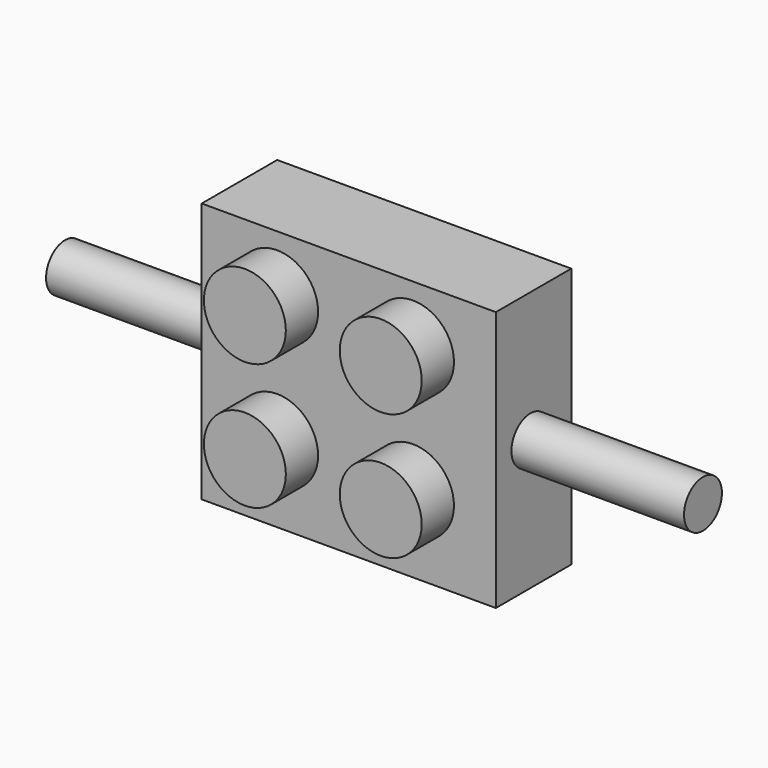
from build123d import *

# Parameters (mm, degrees)
F0_R      = 7.8435703096
F1_DEPTH  = 5.67
F0_R_2    = 7.7757185056
F2_W      = 17.6903378959
F2_H      = 15.67
F3_DEPTH  = 5.67
F4_R      = 1.425
F5_DEPTH  = 10.38
F6_R      = 1.425
F7_DEPTH  = 10.38
F8_R      = 2.465
F9_DEPTH  = 2.425
F10_W     = 12.8629952669
F10_H     = 10.9573621303
F11_DEPTH = 3
F12_R     = 2.75
F12_R_2   = 1.75
F13_DEPTH = 2
F14_R     = 4.345
F14_R_2   = 3.4662678384
F15_DEPTH = 25
F14_R_3   = 3.1273613379
F14_R_4   = 4.1038801884
F14_R_5   = 4.2870364602
F16_DEPTH = 25


with BuildPart() as f1:
    # F0 (on Front) → F1 (new body)
    with BuildSketch(Plane.XZ):
        with Locations((-31.0182443455, 13.5022135742)):
            Circle(F0_R)
    extrude(amount=F1_DEPTH)

    # F14 (on Front) → F15, piece 2 (join)
    with BuildSketch(Plane.XZ):
        with Locations((-31.2459040433, 14.0220327303)):
            Circle(F14_R)
        with Locations((-31.2459040433, 14.0220327303)):
            Circle(F14_R_3, mode=Mode.SUBTRACT)
    extrude(amount=F15_DEPTH)

    # F14 (on Front) → F16 (cut)
    with BuildSketch(Plane.XZ):
        with Locations((27.6749636978, 13.738758862)):
            Circle(F14_R)
        with Locations((27.6749636978, 13.738758862)):
            Circle(F14_R_2, mode=Mode.SUBTRACT)
        with Locations((-30.9626311064, -35.5508103967)):
            Circle(F14_R)
        with Locations((-30.9626311064, -35.5508103967)):
            Circle(F14_R_4, mode=Mode.SUBTRACT)
        with Locations((27.9582366347, -35.5508103967)):
            Circle(F14_R)
        with Locations((27.9582366347, -35.5508103967)):
            Circle(F14_R_5, mode=Mode.SUBTRACT)
        with Locations((-31.2459040433, 14.0220327303)):
            Circle(F14_R)
        with Locations((-31.2459040433, 14.0220327303)):
            Circle(F14_R_3, mode=Mode.SUBTRACT)
    extrude(amount=-F16_DEPTH, mode=Mode.SUBTRACT)


with BuildPart() as f1b:
    # F0 (on Front) → F1, piece 2 (new body)
    with BuildSketch(Plane.XZ):
        with Locations((27.6562659057, 13.5022135742)):
            Circle(F0_R_2)
    extrude(amount=F1_DEPTH)

    # F14 (on Front) → F15 (join)
    with BuildSketch(Plane.XZ):
        with Locations((27.6749636978, 13.738758862)):
            Circle(F14_R)
        with Locations((27.6749636978, 13.738758862)):
            Circle(F14_R_2, mode=Mode.SUBTRACT)
    extrude(amount=F15_DEPTH)


with BuildPart() as f1c:
    # F0 (on Front) → F1, piece 3 (new body)
    with BuildSketch(Plane.XZ):
        with Locations((-31.0182443455, -35.7866174178)):
            Circle(F0_R_2)
    extrude(amount=F1_DEPTH)

    # F14 (on Front) → F15, piece 3 (join)
    with BuildSketch(Plane.XZ):
        with Locations((-30.9626311064, -35.5508103967)):
            Circle(F14_R)
        with Locations((-30.9626311064, -35.5508103967)):
            Circle(F14_R_4, mode=Mode.SUBTRACT)
    extrude(amount=F15_DEPTH)


with BuildPart() as f1d:
    # F0 (on Front) → F1, piece 4 (new body)
    with BuildSketch(Plane.XZ):
        with Locations((27.6562659057, -35.7866174178)):
            Circle(F0_R_2)
    extrude(amount=F1_DEPTH)

    # F14 (on Front) → F15, piece 4 (join)
    with BuildSketch(Plane.XZ):
        with Locations((27.9582366347, -35.5508103967)):
            Circle(F14_R)
        with Locations((27.9582366347, -35.5508103967)):
            Circle(F14_R_5, mode=Mode.SUBTRACT)
    extrude(amount=F15_DEPTH)


with BuildPart() as f3:
    # F2 (on Front) → F3 (new body)
    with BuildSketch(Plane.XZ):
        with Locations((-76.0589055717, 37.1088152751)):
            Rectangle(F2_W, F2_H)
    extrude(amount=F3_DEPTH)

    # F4 (on face) → F5 (join)
    with BuildSketch(Plane(origin=(-84.9040745196, 0, 0), x_dir=(0, -1, 0), z_dir=(-1, 0, 0))):
        with Locations((2.974371193, 37.1088152751)):
            Circle(F4_R)
    extrude(amount=F5_DEPTH)

    # F6 (on face) → F7 (join)
    with BuildSketch(Plane.YZ.offset(-67.2137366238)):
        with Locations((-3.0722431839, 37.1088152751)):
            Circle(F6_R)
    extrude(amount=F7_DEPTH)

    # F8 (on face) → F9 (join)
    with BuildSketch(Plane.XZ.offset(5.67)):
        with Locations((-80.3711495243, 41.4787063429)):
            Circle(F8_R)
        with Locations((-72.1980867, 41.4787063429)):
            Circle(F8_R)
        with Locations((-72.1980867, 33.8693021292)):
            Circle(F8_R)
        with Locations((-80.3711495243, 33.8693021292)):
            Circle(F8_R)
    extrude(amount=F9_DEPTH)

    # F10 (on face) → F11 (cut)
    with BuildSketch(Plane(origin=(0, 0, 0), x_dir=(-1, 0, 0), z_dir=(0, 1, 0))):
        with Locations((76.6844823956, 36.675314419)):
            Rectangle(F10_W, F10_H)
    extrude(amount=-F11_DEPTH, mode=Mode.SUBTRACT)

    # F12 (on face) → F13 (join)
    with BuildSketch(Plane(origin=(0, -3, 0), x_dir=(-1, 0, 0), z_dir=(0, 1, 0))):
        with Locations((76.6844823956, 36.5562103689)):
            Circle(F12_R)
        with Locations((76.6844823956, 36.5562103689)):
            Circle(F12_R_2, mode=Mode.SUBTRACT)
    extrude(amount=F13_DEPTH)


solid = f3.part
